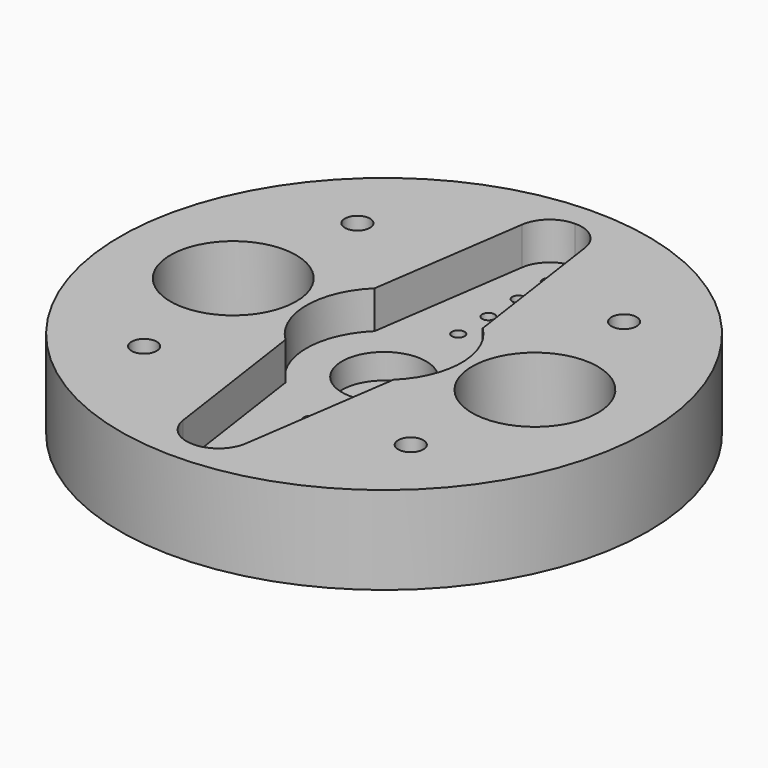
from build123d import *

# Parameters (mm, degrees)
F0_R             = 21
F1_DEPTH         = 7
F3_DEPTH         = 3
F4_R             = 3.35
F5_DEPTH         = 2
F6_R             = 0.5
F7_DEPTH         = 3.4
F8_R             = 5
F9_DEPTH         = 5.5
F13_COPIES_COUNT = 4


# Not quite as in the source:
# - a pattern or mirror of a feature is missing from the dataset's text; its kind, count and spacing are read off the source's solid


with BuildPart() as f1:
    # F0 (on Top) → F1 (new body)
    with BuildSketch(Plane.XY):
        Circle(F0_R)
    extrude(amount=F1_DEPTH)

    # F2 (on face) → F3 (cut)
    with BuildSketch(Plane.XY.offset(7)):
        with BuildLine():
            Line((-2.5, 16.8585155142), (-4.3, 4.4317744753))
            ThreePointArc((-4.3, 4.4317744753), (-6.175, 0), (-4.3, -4.4317744753))
            Line((-4.3, -4.4317744753), (-2.5, -16.8585155142))
            ThreePointArc((-2.5, -16.8585155142), (-1.6521982913, -18.3987898667), (0, -19))
            ThreePointArc((0, -19), (1.6521982913, -18.3987898667), (2.5, -16.8585155142))
            Line((2.5, -16.8585155142), (4.3, -4.4317744753))
            ThreePointArc((4.3, -4.4317744753), (6.175, 0), (4.3, 4.4317744753))
            Line((4.3, 4.4317744753), (2.5, 16.8585155142))
            ThreePointArc((2.5, 16.8585155142), (1.6521982913, 18.3987898667), (0, 19))
            ThreePointArc((0, 19), (-1.6521982913, 18.3987898667), (-2.5, 16.8585155142))
        make_face()
    extrude(amount=-F3_DEPTH, mode=Mode.SUBTRACT)

    # F4 (on face) → F5 (cut)
    with BuildSketch(Plane.XY.offset(4)):
        Circle(F4_R)
    extrude(amount=-F5_DEPTH, mode=Mode.SUBTRACT)

    # F6 (on face) → F7 (cut)
    with BuildSketch(Plane.XY.offset(4)):
        with Locations((0, 7.375)):
            Circle(F6_R)
        with Locations((0, 10.375)):
            Circle(F6_R)
        with Locations((0, 13.375)):
            Circle(F6_R)
        with Locations((0, 16.375)):
            Circle(F6_R)
        with Locations((0, -7.375)):
            Circle(F6_R)
        with Locations((0, -10.375)):
            Circle(F6_R)
        with Locations((0, -13.375)):
            Circle(F6_R)
        with Locations((0, -16.375)):
            Circle(F6_R)
    extrude(amount=-F7_DEPTH, mode=Mode.SUBTRACT)

    # F8 (on face) → F9 (cut, through all)
    with BuildSketch(Plane.XY.offset(7)):
        with Locations((-12, 0)):
            Circle(F8_R)
        with Locations((12, 0)):
            Circle(F8_R)
    extrude(amount=-F9_DEPTH, mode=Mode.SUBTRACT)

    # F12 (on plane+point) → F13 (revolve, cut)
    with BuildSketch(Plane.XZ.offset(10.6066017178)):
        with BuildLine():
            Line((-10.6066017178, 0), (-10.6066017178, 7))
            Line((-10.6066017178, 7), (-11.6066017178, 7.0008294335))
            Line((-11.6066017178, 7.0008294335), (-11.6066017178, 4.2948370387))
            ThreePointArc((-11.6066017178, 4.2948370387), (-13.8675802694, 0.6440169112), (-10.6066017178, -2.15))
            Line((-10.6066017178, -2.15), (-10.6066017178, 0))
        make_face()
    f13 = revolve(axis=Axis((-10.6066017178, -10.6066017178, -1.075), (0, 0, -1)), mode=Mode.SUBTRACT)

    # F13_copies: F13 ×4 about axis
    f13_copies_axis = Axis((0, 0, 0), (0, 0, 1))
    for i in range(1, F13_COPIES_COUNT):
        add(f13.rotate(f13_copies_axis, i * 360 / F13_COPIES_COUNT), mode=Mode.SUBTRACT)


solid = f1.part
